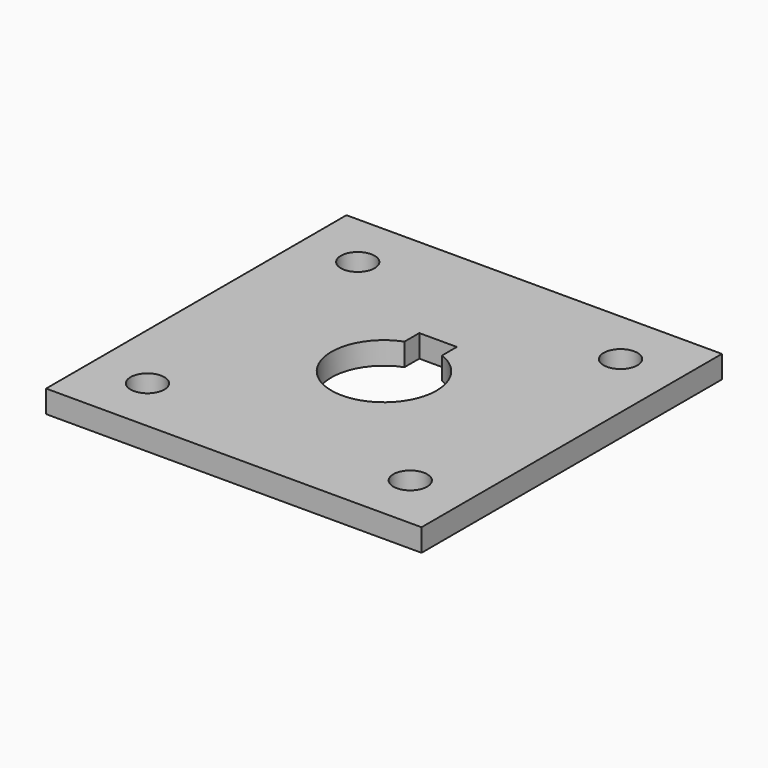
from build123d import *

# Parameters (mm, degrees)
F0_W     = 50
F0_H     = 50
F0_R     = 2
F1_DEPTH = 3
F2_D     = 4.5


# Not quite as in the source:
# - a feature names something its author has since deleted; it is built from what else it names


with BuildPart() as f1:
    # F0 (on Top) → F1 (new body)
    with BuildSketch(Plane.XY):
        with Locations((-50, -49.9732751399)):
            Rectangle(F0_W, F0_H)
        with Locations((-67.5, -67.4732751399)):
            Circle(F0_R, mode=Mode.SUBTRACT)
        with Locations((-32.5, -67.4732751399)):
            Circle(F0_R, mode=Mode.SUBTRACT)
        with Locations((-67.5, -32.4732751399)):
            Circle(F0_R, mode=Mode.SUBTRACT)
        with BuildLine():
            Line((-47.5, -40.9732751399), (-47.5, -43.4349267246))
            ThreePointArc((-47.5, -43.4349267246), (-44.2337187027, -46.0046481733), (-43, -49.9732751399))
            ThreePointArc((-43, -49.9732751399), (-53.9686269666, -55.7395564373), (-52.5, -43.4349267246))
            Line((-52.5, -43.4349267246), (-52.5, -40.9732751399))
            Line((-52.5, -40.9732751399), (-47.5, -40.9732751399))
        make_face(mode=Mode.SUBTRACT)
        with Locations((-32.5, -32.4732751399)):
            Circle(F0_R, mode=Mode.SUBTRACT)
    extrude(amount=F1_DEPTH)

    # F2 (through all)
    with Locations(Plane(origin=(0, 0, 0), x_dir=(1, 0, 0), z_dir=(0, 0, -1))):
        with Locations((-32.5, 32.4732751399), (-32.5, 67.4732751399), (-67.5, 67.4732751399), (-67.5, 32.4732751399)):
            Hole(F2_D / 2)


solid = f1.part
